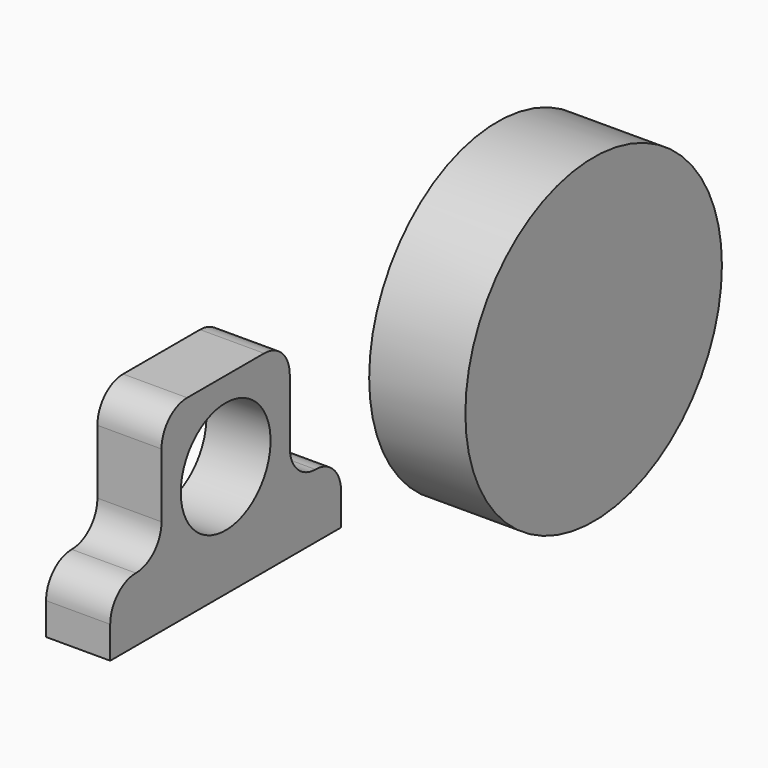
from build123d import *

# Parameters (mm, degrees)
F0_R     = 63.5
F1_DEPTH = 38.1
F2_W     = 63.5
F2_H     = 76.2
F3_DEPTH = 25.4
F5_D     = 44.45
F7_W     = 25.4
F7_H     = 25.4
F8_DEPTH = 25.4
F6_W     = 25.4
F6_H     = 25.4
F9_DEPTH = 25.4
F10_R    = 12.69999


# Not quite as in the source:
# - a fillet or chamfer is up to 0.001 mm smaller than in the source, because OpenCascade refuses the exact size


with BuildPart() as f1:
    # F0 (on Right) → F1 (new body)
    with BuildSketch(Plane.YZ):
        Circle(F0_R)
    extrude(amount=F1_DEPTH)


with BuildPart() as f3:
    # F2 (on Right) → F3 (new body)
    with BuildSketch(Plane.YZ):
        with Locations((-166.2890618503, 12.7576400614)):
            Rectangle(F2_W, F2_H)
    extrude(amount=F3_DEPTH)

    # F5 (through all)
    with Locations(Plane.YZ.offset(25.4)):
        with Locations((-166.2890618503, 19.1076400614)):
            Hole(F5_D / 2)

    # F7 (on face) → F8 (join)
    with BuildSketch(Plane(origin=(0, -134.5390618503, 0), x_dir=(-1, 0, 0), z_dir=(0, 1, 0))):
        with Locations((-12.7, -12.6423599386)):
            Rectangle(F7_W, F7_H)
    extrude(amount=F8_DEPTH)

    # F6 (on face) → F9 (join)
    with BuildSketch(Plane.XZ.offset(198.0390618503)):
        with Locations((12.7, -12.6423599386)):
            Rectangle(F6_W, F6_H)
    extrude(amount=F9_DEPTH)

    # F10 (radius 12.7 in the source; OpenCascade refuses exactly that, so slightly less here)
    f10_edges = [f3.edges().sort_by_distance(p)[0] for p in [
        (12.7, -223.439062, 0.05764),
        (12.7, -198.039062, 0.05764),
        (12.7, -198.039062, 50.85764),
        (12.7, -134.539062, 50.85764),
        (12.7, -134.539062, 0.05764),
        (12.7, -109.139062, 0.05764),
    ]]
    fillet(f10_edges, radius=F10_R)


solid = Compound([f1.part, f3.part])
